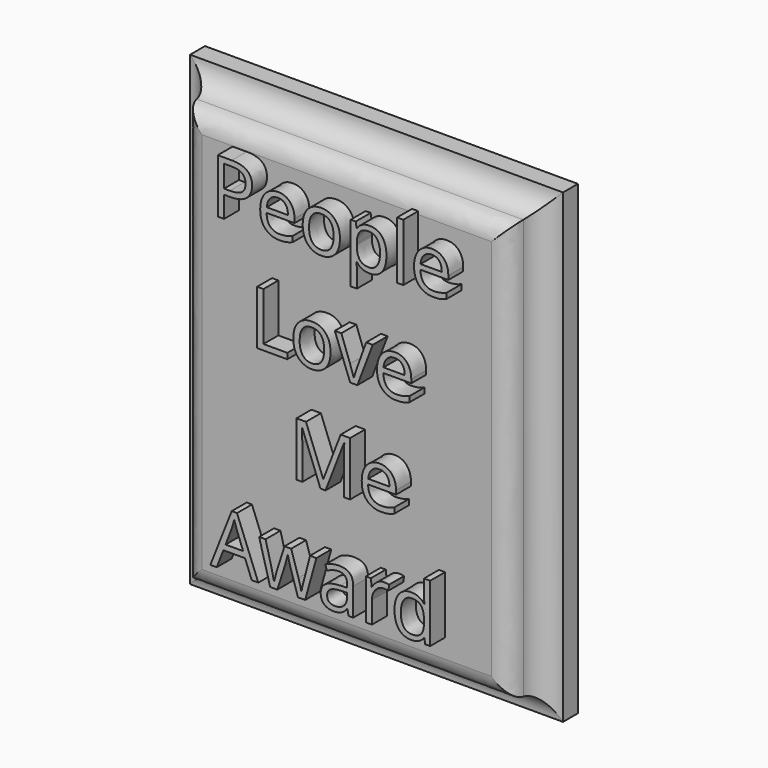
from build123d import *

# Parameters (mm, degrees)
F0_W         = 101.6
F0_H         = 127
F1_DEPTH     = 15.24
F2_W         = 101.6
F2_H         = 127
F2_W_2       = 88.9
F2_H_2       = 114.3
F3_DEPTH     = 10.16
F4_R         = 6.34999
F5_R         = 5.08
F6_TEXT_SIZE = 20.639407262
F7_DEPTH     = 5.08


# Not quite as in the source:
# - a fillet or chamfer is up to 0.001 mm smaller than in the source, because OpenCascade refuses the exact size
# - Text() gives the source's letters only with a copy of the font that has no kerning and outlines rounded to 1/6400 em; it was checked with that copy


with BuildPart() as f1:
    # F0 (on Front) → F1 (new body)
    with BuildSketch(Plane.XZ):
        with Locations((-50.8, 63.5)):
            Rectangle(F0_W, F0_H)
    extrude(amount=F1_DEPTH)

    # F2 (on face) → F3 (cut)
    with BuildSketch(Plane.XZ.offset(15.24)):
        with Locations((-50.8, 63.5)):
            Rectangle(F2_W, F2_H)
        with Locations((-50.8, 63.5)):
            Rectangle(F2_W_2, F2_H_2, mode=Mode.SUBTRACT)
    extrude(amount=-F3_DEPTH, mode=Mode.SUBTRACT)

    # F4 (radius 6.35 in the source; OpenCascade refuses exactly that, so slightly less here)
    f4_edges = [f1.edges().sort_by_distance(p)[0] for p in [
        (-50.8, -5.08, 120.65),
        (-6.35, -5.08, 63.5),
        (-95.25, -5.08, 63.5),
        (-50.8, -5.08, 6.35),
    ]]
    fillet(f4_edges, radius=F4_R)

    # F5
    f5_edges = [f1.edges().sort_by_distance(p)[0] for p in [
        (-6.35, -15.24, 63.5),
        (-50.8, -15.24, 6.35),
        (-95.25, -15.24, 63.5),
        (-50.8, -15.24, 120.65),
    ]]
    fillet(f5_edges, radius=F5_R)

    # F6 (on face) → F7 (join)
    with BuildSketch(Plane.XZ.offset(15.24)):
        with Locations((-83.8907746743, 100.7804014457)):
            Text('People', F6_TEXT_SIZE, font='Open Sans', text_align=(TextAlign.LEFT, TextAlign.BOTTOM))
        with Locations((-73.1647327128, 72.7108075693)):
            Text('Love', F6_TEXT_SIZE, font='Open Sans', text_align=(TextAlign.LEFT, TextAlign.BOTTOM))
        with Locations((-62.4386907513, 44.641213693)):
            Text('Me', F6_TEXT_SIZE, font='Open Sans', text_align=(TextAlign.LEFT, TextAlign.BOTTOM))
        with Locations((-83.8907746743, 16.5716198166)):
            Text('Award', F6_TEXT_SIZE, font='Open Sans', text_align=(TextAlign.LEFT, TextAlign.BOTTOM))
    extrude(amount=F7_DEPTH)


solid = f1.part
